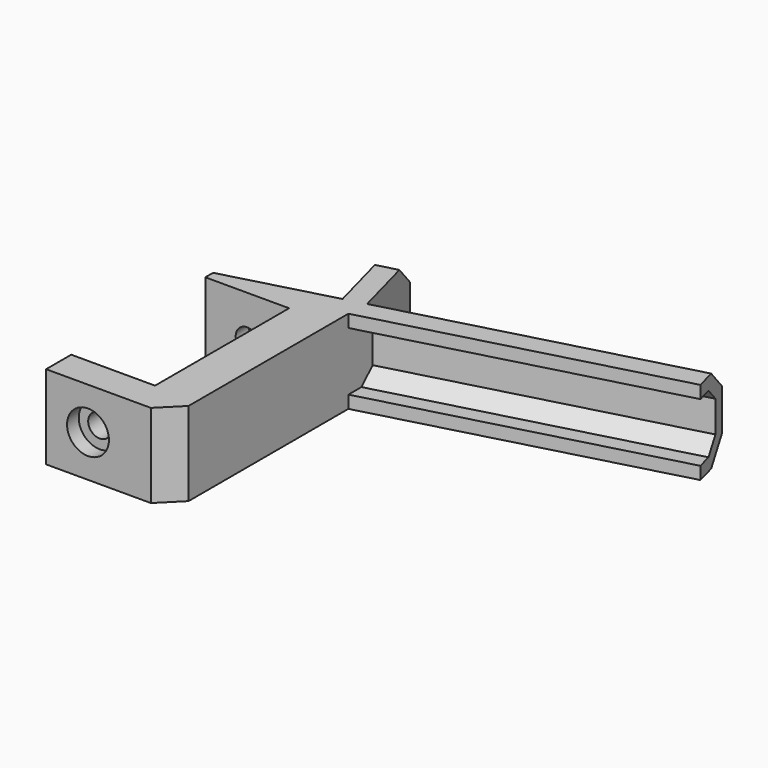
from build123d import *

# Parameters (mm, degrees)
F1_DEPTH  = 20
F2_R      = 2.75
F3_DEPTH  = 80.8829045103
F5_R      = 5
F6_DEPTH  = 29.3829045103
F7_R      = 5
F8_DEPTH  = 3.5
F9_SIZE   = 4.99999
F11_REACH = 132.6751363952


# Not quite as in the source:
# - a fillet or chamfer is up to 0.001 mm smaller than in the source, because OpenCascade refuses the exact size


with BuildPart() as f1:
    # F0 (on Top) → F1 (new body)
    with BuildSketch(Plane.XY):
        Polygon((24.1481456572, 6.4704761276), (0, 0), (0, -7.5), (20, -7.5), (20, -47.5), (0, -47.5), (0, -55), (25, -55), (30, -50), (30, -2.3142860312), (99.1807730799, 16.2226462474), (96.5925826289, 25.8819045103), (28.9777747887, 7.7645713531), (25.0954891121, 22.2534587474), (20.2658599807, 20.9593635219), align=None)
    extrude(amount=F1_DEPTH)

    # F2 (on face) → F3 (cut, through all)
    with BuildSketch(Plane.XZ.offset(55)):
        with Locations((10, 10)):
            Circle(F2_R)
    extrude(amount=-F3_DEPTH, mode=Mode.SUBTRACT)

    # F5 (on offset) → F6 (cut, through all)
    with BuildSketch(Plane.XZ.offset(3.5)):
        with Locations((10, 10)):
            Circle(F5_R)
    extrude(amount=-F6_DEPTH, mode=Mode.SUBTRACT)

    # F7 (on face) → F8 (cut)
    with BuildSketch(Plane.XZ.offset(55)):
        with Locations((10, 10)):
            Circle(F7_R)
    extrude(amount=-F8_DEPTH, mode=Mode.SUBTRACT)

    # F9 (size 5 in the source; OpenCascade refuses exactly that, so slightly less here)
    f9_edges = [f1.edges().sort_by_distance(p)[0] for p in [
        (62.785179, 16.823238, 0),
        (62.785179, 16.823238, 20),
        (12.074073, 3.235238, 20),
        (12.074073, 3.235238, 0),
        (22.680675, 21.606411, 20),
        (22.680675, 21.606411, 0),
    ]]
    chamfer(f9_edges, length=F9_SIZE)

    f11_end = Plane(origin=(30, -26.1571430156, 10), x_dir=(0, 0, 1), z_dir=(1, 0, 0))
    # F10 (on face) → F11 (cut, up to a plane its end follows)
    with BuildSketch(Plane(origin=(96.5925826289, 25.8819045103, 0), x_dir=(-0.2588190451, 0.9659258263, 0), z_dir=(0.9659258263, 0.2588190451, 0))):
        Polygon((-3, 13.7573593129), (-6.2426406871, 17), (-15, 17), (-15, 3), (-6.2426406871, 3), (-3, 6.2426406871), align=None)
    f11_long = extrude(amount=-F11_REACH, mode=Mode.PRIVATE)
    add(split(f11_long, bisect_by=f11_end, keep=Keep.TOP, mode=Mode.PRIVATE), mode=Mode.SUBTRACT)


solid = f1.part
